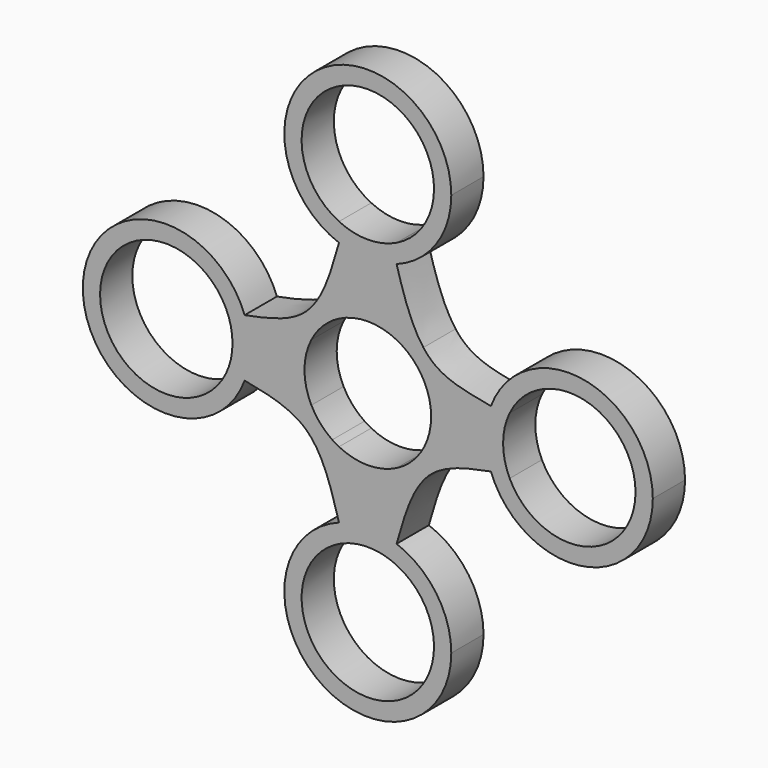
from build123d import *

# Parameters (mm, degrees)
F1_DEPTH = 7


with BuildPart() as f1:
    # F0 (on Front) → F1 (new body)
    with BuildSketch(Plane.XZ):
        with BuildLine():
            ThreePointArc((9.7979589711, 5), (10.695268783, 2.5712303784), (11, 0))
            ThreePointArc((11, 0), (10.695268783, -2.5712303784), (9.7979589711, -5))
            Line((9.7979589711, -5), (13.0766968306, -5))
            ThreePointArc((13.0766968306, -5), (13.7672392953, -2.542267135), (14, 0))
            ThreePointArc((14, 0), (13.7672392953, 2.542267135), (13.0766968306, 5))
            Line((13.0766968306, 5), (9.7979589711, 5))
        make_face()
        with BuildLine():
            ThreePointArc((5, 9.7979589711), (7.7781745931, 7.7781745931), (9.7979589711, 5))
            Line((9.7979589711, 5), (13.0766968306, 5))
            ThreePointArc((13.0766968306, 5), (12.1766661067, 6.9086035149), (11, 8.6602540378))
            add(Edge.make_bspline(
                [(11, 8.6602540378), (10.5165329788, 9.0943534866), (10.069073109, 9.5914231948), (9.6528657807, 10.1401273276)],
                knots=[0.4694223133, 0.4694223133, 0.4694223133, 0.4694223133, 0.5544432682, 0.5544432682, 0.5544432682, 0.5544432682], degree=3))
            ThreePointArc((9.6528657807, 10.1401273276), (7.4721134232, 11.8392365037), (5, 13.0766968306))
            Line((5, 13.0766968306), (5, 9.7979589711))
        make_face()
        with BuildLine():
            Line((13.0766968306, -5), (9.7979589711, -5))
            ThreePointArc((9.7979589711, -5), (8.2425593884, -7.2842442798), (6.166922169, -9.1087359694))
            Line((6.166922169, -9.1087359694), (10.6316004928, -9.1087359694))
            ThreePointArc((10.6316004928, -9.1087359694), (12.0308465334, -7.1595203533), (13.0766968306, -5))
        make_face()
        with BuildLine():
            ThreePointArc((-5, 9.7979589711), (0, 11), (5, 9.7979589711))
            Line((5, 9.7979589711), (5, 13.0766968306))
            ThreePointArc((5, 13.0766968306), (0, 14), (-5, 13.0766968306))
            Line((-5, 13.0766968306), (-5, 9.7979589711))
        make_face()
        with BuildLine():
            ThreePointArc((11, 8.6602540378), (12.1766661067, 6.9086035149), (13.0766968306, 5))
            Line((13.0766968306, 5), (21.3893424112, 5))
            add(Edge.make_bspline(
                [(21.3893424112, 5), (17.4363397181, 5.7863082094), (13.6693443727, 6.2634805868), (11, 8.6602540378)],
                knots=[0, 0, 0, 0, 0.4694223133, 0.4694223133, 0.4694223133, 0.4694223133], degree=3))
        make_face()
        with BuildLine():
            Line((21.3893424112, 5), (13.0766968306, 5))
            ThreePointArc((13.0766968306, 5), (13.7672392953, 2.542267135), (14, 0))
            ThreePointArc((14, 0), (13.7672392953, -2.542267135), (13.0766968306, -5))
            Line((13.0766968306, -5), (21.3893424112, -5))
            ThreePointArc((21.3893424112, -5), (20.5, 0), (21.3893424112, 5))
        make_face()
        with BuildLine():
            Line((10.6316004928, -9.1087359694), (6.166922169, -9.1087359694))
            ThreePointArc((6.166922169, -9.1087359694), (5.5940856955, -9.4713359792), (5, -9.7979589711))
            Line((5, -9.7979589711), (5, -13.0766968306))
            ThreePointArc((5, -13.0766968306), (7.5360949415, -11.7986131826), (9.7620843684, -10.0350241048))
            add(Edge.make_bspline(
                [(10.6316004928, -9.1087359694), (10.3251306555, -9.395868762), (10.035894736, -9.7054154416), (9.7620843684, -10.0350241048)],
                knots=[0.4800426808, 0.4800426808, 0.4800426808, 0.4800426808, 0.5346021309, 0.5346021309, 0.5346021309, 0.5346021309], degree=3))
        make_face()
        with BuildLine():
            Line((21.3893424112, -5), (13.0766968306, -5))
            ThreePointArc((13.0766968306, -5), (12.0308465334, -7.1595203533), (10.6316004928, -9.1087359694))
            add(Edge.make_bspline(
                [(21.3893424112, -5), (17.3587127001, -5.7911954717), (13.3280829889, -6.5823909435), (10.6316004928, -9.1087359694)],
                knots=[0, 0, 0, 0, 0.4800426808, 0.4800426808, 0.4800426808, 0.4800426808], degree=3))
        make_face()
        with BuildLine():
            ThreePointArc((-9.7979589711, 5), (-7.7781745931, 7.7781745931), (-5, 9.7979589711))
            Line((-5, 9.7979589711), (-5, 13.0766968306))
            ThreePointArc((-5, 13.0766968306), (-7.5358238199, 11.798786351), (-9.7616231696, 10.0354727389))
            add(Edge.make_bspline(
                [(-9.7616231696, 10.0354727389), (-10.0355905847, 9.7057125821), (-10.3249817585, 9.3960175313), (-10.6316004928, 9.1087359694)],
                knots=[0.4653704717, 0.4653704717, 0.4653704717, 0.4653704717, 0.5199573192, 0.5199573192, 0.5199573192, 0.5199573192], degree=3))
            ThreePointArc((-10.6316004928, 9.1087359694), (-12.0308465334, 7.1595203533), (-13.0766968306, 5))
            Line((-13.0766968306, 5), (-9.7979589711, 5))
        make_face()
        with BuildLine():
            ThreePointArc((-5, 13.0766968306), (0, 14), (5, 13.0766968306))
            Line((5, 13.0766968306), (5, 21.3893424112))
            ThreePointArc((5, 21.3893424112), (0, 20.5), (-5, 21.3893424112))
            Line((-5, 21.3893424112), (-5, 13.0766968306))
        make_face()
        with BuildLine():
            Line((5, 21.3893424112), (5, 13.0766968306))
            ThreePointArc((5, 13.0766968306), (7.4721134232, 11.8392365037), (9.6528657807, 10.1401273276))
            add(Edge.make_bspline(
                [(9.6528657807, 10.1401273276), (7.4717096508, 13.0156398459), (6.1488540964, 17.3092084385), (5, 21.3893424112)],
                knots=[0.5544432682, 0.5544432682, 0.5544432682, 0.5544432682, 1, 1, 1, 1], degree=3))
        make_face()
        with BuildLine():
            ThreePointArc((49.5, 0), (37.5392385632, 14.2759331576), (21.3893424112, 5))
            Line((21.3893424112, 5), (24.6438424114, 5))
            ThreePointArc((24.6438424114, 5), (37.5645845405, 11.2103927734), (46.5, 0))
            ThreePointArc((46.5, 0), (37.5645845405, -11.2103927734), (24.6438424114, -5))
            Line((24.6438424114, -5), (21.3893424112, -5))
            ThreePointArc((21.3893424112, -5), (37.5392385632, -14.2759331576), (49.5, 0))
        make_face()
        with BuildLine():
            Line((24.6438424114, 5), (21.3893424112, 5))
            ThreePointArc((21.3893424112, 5), (20.5, 0), (21.3893424112, -5))
            Line((21.3893424112, -5), (24.6438424114, -5))
            ThreePointArc((24.6438424114, -5), (23.5, 0), (24.6438424114, 5))
        make_face()
        with BuildLine():
            Line((5, -13.0766968306), (5, -9.7979589711))
            ThreePointArc((5, -9.7979589711), (0, -11), (-5, -9.7979589711))
            Line((-5, -9.7979589711), (-5, -13.0766968306))
            ThreePointArc((-5, -13.0766968306), (0, -14), (5, -13.0766968306))
        make_face()
        with BuildLine():
            ThreePointArc((-9.7979589711, -5), (-11, 0), (-9.7979589711, 5))
            Line((-9.7979589711, 5), (-13.0766968306, 5))
            ThreePointArc((-13.0766968306, 5), (-14, 0), (-13.0766968306, -5))
            Line((-13.0766968306, -5), (-9.7979589711, -5))
        make_face()
        with BuildLine():
            ThreePointArc((-9.7616231696, 10.0354727389), (-7.5358238199, 11.798786351), (-5, 13.0766968306))
            Line((-5, 13.0766968306), (-5, 21.3893424112))
            add(Edge.make_bspline(
                [(-5, 21.3893424112), (-6.2113181827, 17.1164504192), (-7.4259626407, 12.8467843762), (-9.7616231696, 10.0354727389)],
                knots=[0, 0, 0, 0, 0.4653704717, 0.4653704717, 0.4653704717, 0.4653704717], degree=3))
        make_face()
        with BuildLine():
            ThreePointArc((-5, 21.3893424112), (0, 20.5), (5, 21.3893424112))
            Line((5, 21.3893424112), (5, 24.6438424114))
            ThreePointArc((5, 24.6438424114), (0, 23.5), (-5, 24.6438424114))
            Line((-5, 24.6438424114), (-5, 21.3893424112))
        make_face()
        with BuildLine():
            Line((5, 24.6438424114), (5, 21.3893424112))
            ThreePointArc((5, 21.3893424112), (11.8901219506, 26.7009036637), (14.5, 35))
            ThreePointArc((14.5, 35), (-8.2990963363, 46.8901219506), (-5, 21.3893424112))
            Line((-5, 21.3893424112), (-5, 24.6438424114))
            ThreePointArc((-5, 24.6438424114), (-6.1135096303, 44.7403798694), (11.5, 35))
            ThreePointArc((11.5, 35), (9.7403798694, 28.8864903697), (5, 24.6438424114))
        make_face()
        with BuildLine():
            Line((-5, -13.0766968306), (-5, -9.7979589711))
            ThreePointArc((-5, -9.7979589711), (-5.5940856955, -9.4713359792), (-6.166922169, -9.1087359694))
            Line((-6.166922169, -9.1087359694), (-10.6316004928, -9.1087359694))
            add(Edge.make_bspline(
                [(-10.6316004928, -9.1087359694), (-10.3251306555, -9.395868762), (-10.035894736, -9.7054154416), (-9.7620843684, -10.0350241048)],
                knots=[0.4800426808, 0.4800426808, 0.4800426808, 0.4800426808, 0.5346021309, 0.5346021309, 0.5346021309, 0.5346021309], degree=3))
            ThreePointArc((-9.7620843684, -10.0350241048), (-7.5360949415, -11.7986131826), (-5, -13.0766968306))
        make_face()
        with BuildLine():
            ThreePointArc((9.7620843684, -10.0350241048), (7.5360949415, -11.7986131826), (5, -13.0766968306))
            Line((5, -13.0766968306), (5, -21.3893424112))
            add(Edge.make_bspline(
                [(9.7620843684, -10.0350241048), (7.4264530295, -12.8466207961), (6.2132265148, -17.1179816036), (5, -21.3893424112)],
                knots=[0.5346021309, 0.5346021309, 0.5346021309, 0.5346021309, 1, 1, 1, 1], degree=3))
        make_face()
        with BuildLine():
            Line((5, -21.3893424112), (5, -13.0766968306))
            ThreePointArc((5, -13.0766968306), (0, -14), (-5, -13.0766968306))
            Line((-5, -13.0766968306), (-5, -21.3893424112))
            ThreePointArc((-5, -21.3893424112), (0, -20.5), (5, -21.3893424112))
        make_face()
        with BuildLine():
            ThreePointArc((-6.166922169, -9.1087359694), (-8.2425593884, -7.2842442798), (-9.7979589711, -5))
            Line((-9.7979589711, -5), (-13.0766968306, -5))
            ThreePointArc((-13.0766968306, -5), (-12.0308465334, -7.1595203533), (-10.6316004928, -9.1087359694))
            Line((-10.6316004928, -9.1087359694), (-6.166922169, -9.1087359694))
        make_face()
        with BuildLine():
            ThreePointArc((-13.0766968306, -5), (-14, 0), (-13.0766968306, 5))
            Line((-13.0766968306, 5), (-21.3893424112, 5))
            ThreePointArc((-21.3893424112, 5), (-20.7240668424, 2.5392385632), (-20.5, 0))
            ThreePointArc((-20.5, 0), (-20.7240668424, -2.5392385632), (-21.3893424112, -5))
            Line((-21.3893424112, -5), (-13.0766968306, -5))
        make_face()
        with BuildLine():
            Line((-21.3893424112, 5), (-13.0766968306, 5))
            ThreePointArc((-13.0766968306, 5), (-12.0308465334, 7.1595203533), (-10.6316004928, 9.1087359694))
            add(Edge.make_bspline(
                [(-10.6316004928, 9.1087359694), (-13.3280390276, 6.5823506348), (-17.3567942358, 5.789342747), (-21.3893424112, 5)],
                knots=[0.5199573192, 0.5199573192, 0.5199573192, 0.5199573192, 1, 1, 1, 1], degree=3))
        make_face()
        with BuildLine():
            Line((-5, -21.3893424112), (-5, -13.0766968306))
            ThreePointArc((-5, -13.0766968306), (-7.5360949415, -11.7986131826), (-9.7620843684, -10.0350241048))
            add(Edge.make_bspline(
                [(-9.7620843684, -10.0350241048), (-7.4264530295, -12.8466207961), (-6.2132265148, -17.1179816036), (-5, -21.3893424112)],
                knots=[0.5346021309, 0.5346021309, 0.5346021309, 0.5346021309, 1, 1, 1, 1], degree=3))
        make_face()
        with BuildLine():
            ThreePointArc((14.5, -35), (11.8901219506, -26.7009036637), (5, -21.3893424112))
            Line((5, -21.3893424112), (5, -24.6438424114))
            ThreePointArc((5, -24.6438424114), (9.7403798694, -28.8864903697), (11.5, -35))
            ThreePointArc((11.5, -35), (-6.1135096303, -44.7403798694), (-5, -24.6438424114))
            Line((-5, -24.6438424114), (-5, -21.3893424112))
            ThreePointArc((-5, -21.3893424112), (-8.2990963363, -46.8901219506), (14.5, -35))
        make_face()
        with BuildLine():
            Line((5, -24.6438424114), (5, -21.3893424112))
            ThreePointArc((5, -21.3893424112), (0, -20.5), (-5, -21.3893424112))
            Line((-5, -21.3893424112), (-5, -24.6438424114))
            ThreePointArc((-5, -24.6438424114), (0, -23.5), (5, -24.6438424114))
        make_face()
        with BuildLine():
            ThreePointArc((-10.6316004928, -9.1087359694), (-12.0308465334, -7.1595203533), (-13.0766968306, -5))
            Line((-13.0766968306, -5), (-21.3893424112, -5))
            add(Edge.make_bspline(
                [(-21.3893424112, -5), (-17.3587127001, -5.7911954717), (-13.3280829889, -6.5823909435), (-10.6316004928, -9.1087359694)],
                knots=[0, 0, 0, 0, 0.4800426808, 0.4800426808, 0.4800426808, 0.4800426808], degree=3))
        make_face()
        with BuildLine():
            ThreePointArc((-20.5, 0), (-20.7240668424, 2.5392385632), (-21.3893424112, 5))
            Line((-21.3893424112, 5), (-24.6438424114, 5))
            ThreePointArc((-24.6438424114, 5), (-23.7896072266, 2.5645845405), (-23.5, 0))
            ThreePointArc((-23.5, 0), (-23.7896072266, -2.5645845405), (-24.6438424114, -5))
            Line((-24.6438424114, -5), (-21.3893424112, -5))
            ThreePointArc((-21.3893424112, -5), (-20.7240668424, -2.5392385632), (-20.5, 0))
        make_face()
        with BuildLine():
            Line((-24.6438424114, 5), (-21.3893424112, 5))
            ThreePointArc((-21.3893424112, 5), (-49.5, 0), (-21.3893424112, -5))
            Line((-21.3893424112, -5), (-24.6438424114, -5))
            ThreePointArc((-24.6438424114, -5), (-46.5, 0), (-24.6438424114, 5))
        make_face()
    extrude(amount=F1_DEPTH)


solid = f1.part
